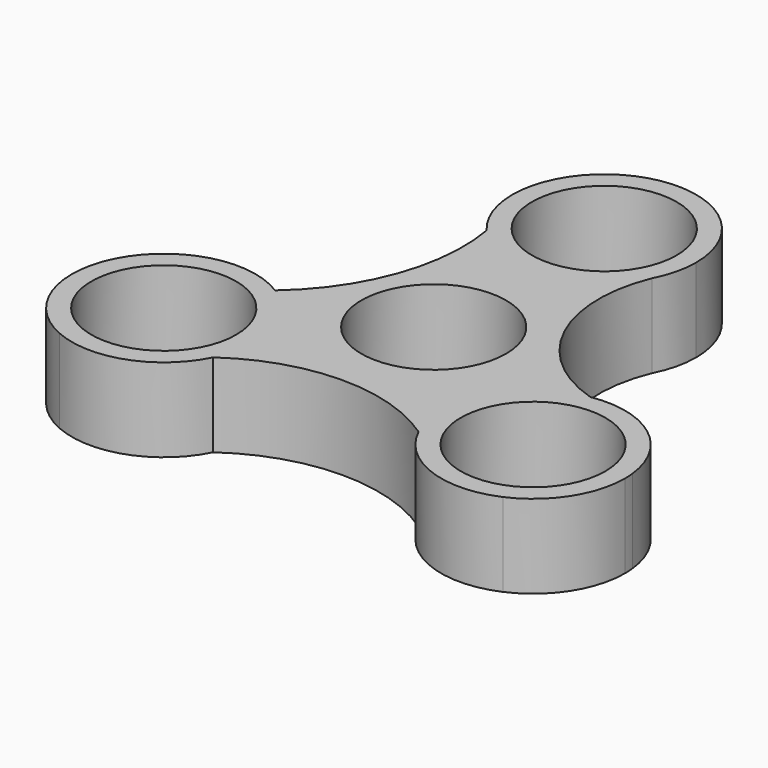
from build123d import *

# Parameters (mm, degrees)
F0_R     = 10.9982
F0_R_2   = 13.97
F1_DEPTH = 12.7


with BuildPart() as f1:
    # F0 (on Top) → F1 (new body)
    with BuildSketch(Plane.XY):
        with BuildLine():
            ThreePointArc((13.97, 32.4071533978), (12.4598818148, 38.7247672797), (8.2560064193, 43.6765481466))
            ThreePointArc((8.2560064193, 43.6765481466), (0, 44.45), (-8.2560064193, 43.6765481466))
            ThreePointArc((-8.2560064193, 43.6765481466), (-13.8783328045, 34.0048951062), (-10.600858317, 23.3086533597))
            ThreePointArc((-10.600858317, 23.3086533597), (1.6096047371, 18.5301914612), (12.4020690853, 25.9767893021))
            ThreePointArc((12.4020690853, 25.9767893021), (13.5723580324, 29.097773178), (13.97, 32.4071533978))
        make_face()
        with Locations((0, 32.4071533978)):
            Circle(F0_R, mode=Mode.SUBTRACT)
        with BuildLine():
            ThreePointArc((-8.2560064193, 43.6765481466), (0, 44.45), (8.2560064193, 43.6765481466))
            ThreePointArc((8.2560064193, 43.6765481466), (0, 46.3771533978), (-8.2560064193, 43.6765481466))
        make_face()
        with BuildLine():
            ThreePointArc((42.0354181068, -16.2035766989), (42.0147992276, -15.4448499046), (41.9530034542, -14.6883627804))
            ThreePointArc((41.9530034542, -14.6883627804), (38.4948291982, -22.225), (33.696997035, -28.9881853662))
            ThreePointArc((33.696997035, -28.9881853662), (39.7665731273, -23.8353439377), (42.0354181068, -16.2035766989))
        make_face()
        with BuildLine():
            ThreePointArc((33.696997035, -28.9881853662), (38.4948291982, -22.225), (41.9530034542, -14.6883627804))
            ThreePointArc((41.9530034542, -14.6883627804), (36.4931838712, -5.0620478891), (25.7444185967, -2.4277333028))
            ThreePointArc((25.7444185967, -2.4277333028), (15.6881084253, -9.7256831332), (15.4233394109, -22.1482168264))
            ThreePointArc((15.4233394109, -22.1482168264), (23.1681669233, -29.287071295), (33.696997035, -28.9881853662))
        make_face()
        with Locations((28.0654181068, -16.2035766989)):
            Circle(F0_R, mode=Mode.SUBTRACT)
        with BuildLine():
            ThreePointArc((15.4233394109, -22.1482168264), (15.6881084253, -9.7256831332), (25.7444185967, -2.4277333028))
            ThreePointArc((25.7444185967, -2.4277333028), (12.8005092874, 8.8280600033), (12.4020690853, 25.9767893021))
            ThreePointArc((12.4020690853, 25.9767893021), (1.6096047371, 18.5301914612), (-10.600858317, 23.3086533597))
            ThreePointArc((-10.600858317, 23.3086533597), (-11.9457670792, 8.1377589695), (-20.5888732511, -4.4026370321))
            ThreePointArc((-20.5888732511, -4.4026370321), (-15.8259689437, -9.4688321468), (-14.0954181068, -16.2035766989))
            ThreePointArc((-14.0954181068, -16.2035766989), (-14.4683809608, -19.410051531), (-15.5673552362, -22.4453172))
            ThreePointArc((-15.5673552362, -22.4453172), (-0.1187696418, -17.419026699), (15.4233394109, -22.1482168264))
        make_face()
        Circle(F0_R_2, mode=Mode.SUBTRACT)
        with BuildLine():
            ThreePointArc((-20.5888732511, -4.4026370321), (-34.1254839966, -3.6164204906), (-41.9530034542, -14.6883627804))
            ThreePointArc((-41.9530034542, -14.6883627804), (-38.4948291982, -22.225), (-33.696997035, -28.9881853662))
            ThreePointArc((-33.696997035, -28.9881853662), (-23.3231157764, -29.3440283124), (-15.5673552362, -22.4453172))
            ThreePointArc((-15.5673552362, -22.4453172), (-14.4683809608, -19.410051531), (-14.0954181068, -16.2035766989))
            ThreePointArc((-14.0954181068, -16.2035766989), (-15.8259689437, -9.4688321468), (-20.5888732511, -4.4026370321))
        make_face()
        with Locations((-28.0654181068, -16.2035766989)):
            Circle(F0_R, mode=Mode.SUBTRACT)
        with BuildLine():
            ThreePointArc((-33.696997035, -28.9881853662), (-38.4948291982, -22.225), (-41.9530034542, -14.6883627804))
            ThreePointArc((-41.9530034542, -14.6883627804), (-40.1637929977, -23.1885766989), (-33.696997035, -28.9881853662))
        make_face()
        Circle(F0_R_2)
        Circle(F0_R, mode=Mode.SUBTRACT)
    extrude(amount=F1_DEPTH)


solid = f1.part
